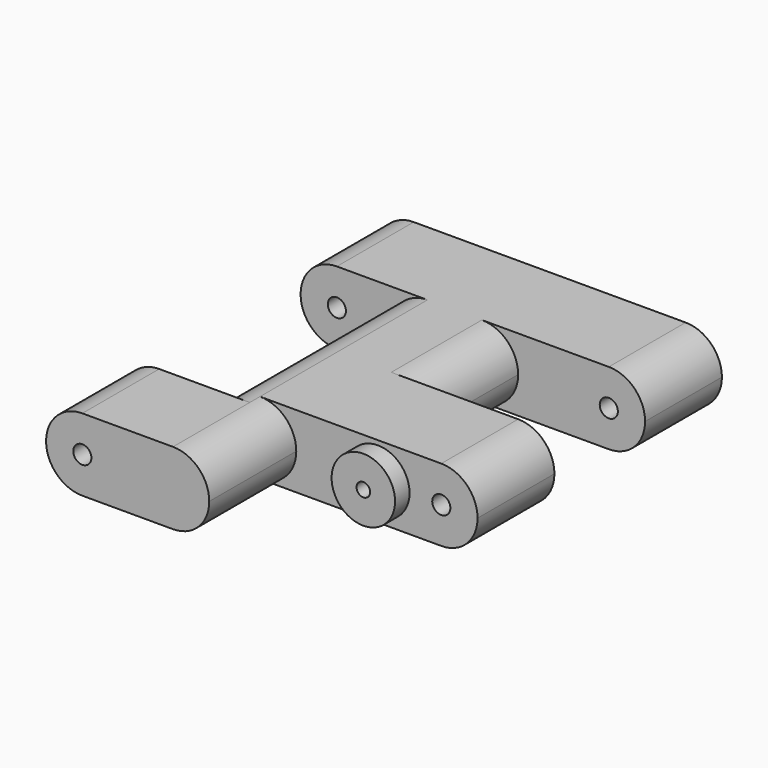
from build123d import *

# Parameters (mm, degrees)
F1_DEPTH = 8
F2_R     = 3.99999
F3_R     = 1
F4_DEPTH = 60
F6_R     = 3.99999
F5_R     = 3.5
F7_DEPTH = 2
F8_R     = 0.75
F9_DEPTH = 12


# Not quite as in the source:
# - a fillet or chamfer is up to 0.001 mm smaller than in the source, because OpenCascade refuses the exact size


with BuildPart() as f1:
    # F0 (on Top) → F1 (new body)
    with BuildSketch(Plane.XY):
        Polygon((-9.9077894302, -1.920078908), (-9.9077894302, -12.520078908), (8.0922105698, -12.520078908), (8.0922105698, -0.520078908), (28.0922105698, -0.520078908), (28.0922105698, 10.079921092), (14.0922105698, 10.079921092), (14.0922105698, 22.579921092), (28.0922105698, 22.579921092), (28.0922105698, 33.179921092), (-9.9077894302, 33.179921092), (-9.9077894302, 22.579921092), (0.0922105698, 22.579921092), (0.0922105698, -1.920078908), align=None)
    extrude(amount=F1_DEPTH)

    # F2 (radius 4 in the source; OpenCascade refuses exactly that, so slightly less here)
    f2_edges = [f1.edges().sort_by_distance(p)[0] for p in [
        (-9.907789, -7.220079, 8),
        (-9.907789, -7.220079, 0),
        (8.092211, -6.520079, 8),
        (8.092211, -6.520079, 0),
        (28.092211, 4.779921, 8),
        (28.092211, 4.779921, 0),
        (28.092211, 27.879921, 8),
        (28.092211, 27.879921, 0),
        (-9.907789, 27.879921, 8),
        (-9.907789, 27.879921, 0),
    ]]
    fillet(f2_edges, radius=F2_R)

    # F3 (on face) → F4 (cut)
    with BuildSketch(Plane(origin=(0, 33.179921092, 0), x_dir=(-1, 0, 0), z_dir=(0, 1, 0))):
        with Locations((-24.0922105698, 4)):
            Circle(F3_R)
        with Locations((5.9077894302, 4)):
            Circle(F3_R)
    extrude(amount=-F4_DEPTH, mode=Mode.SUBTRACT)

    # F6 (radius 4 in the source; OpenCascade refuses exactly that, so slightly less here)
    f6_edges = [f1.edges().sort_by_distance(p)[0] for p in [
        (0.092211, 10.329921, 8),
        (0.092211, 10.329921, 0),
        (14.092211, 16.329921, 8),
        (14.092211, 16.329921, 0),
    ]]
    fillet(f6_edges, radius=F6_R)

    # F5 (on face) → F7 (join)
    with BuildSketch(Plane.XZ.offset(0.520078908)):
        with Locations((17.0922105698, 4)):
            Circle(F5_R)
    extrude(amount=F7_DEPTH)

    # F8 (on face) → F9 (cut)
    with BuildSketch(Plane.XZ.offset(2.520078908)):
        with Locations((17.0922105698, 4)):
            Circle(F8_R)
    extrude(amount=-F9_DEPTH, mode=Mode.SUBTRACT)


solid = f1.part
